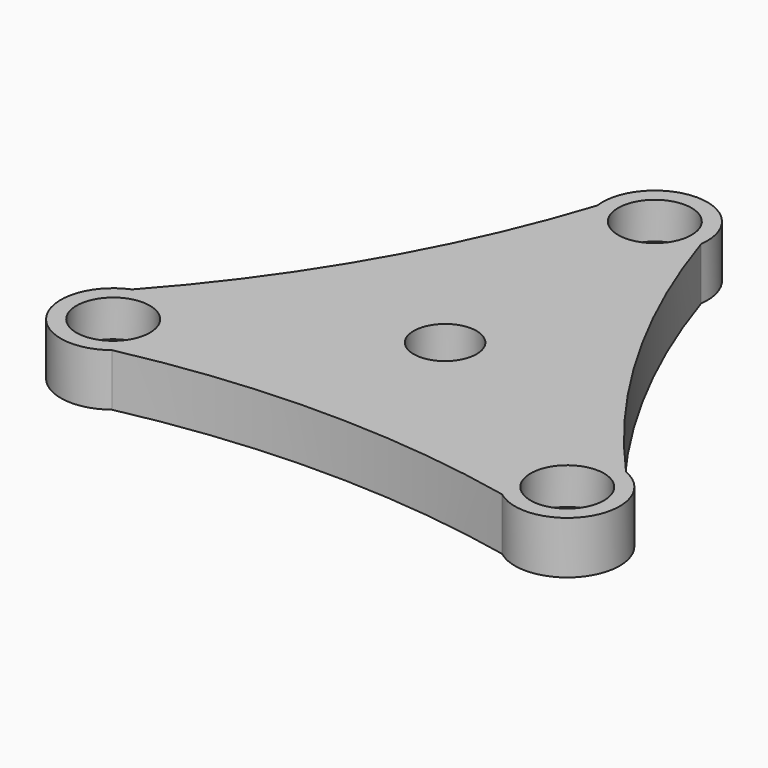
from build123d import *

# Parameters (mm, degrees)
F1_R     = 7
F1_R_2   = 6
F1_R_3   = 5
F2_DEPTH = 3
F3_DEPTH = 10


# Not quite as in the source:
# - a feature of the source that left no trace in its solid (it failed there, or was rolled back) is left out


with BuildPart() as f2:
    # F1 (on Top) → F2 (new body)
    with BuildSketch(Plane.XY):
        with BuildLine():
            ThreePointArc((9.9107145783, 48.6666821283), (0, 60), (-9.9107145783, 48.6666821283))
            ThreePointArc((-9.9107145783, 48.6666821283), (-25.1057988762, 14.4948397394), (-47.1019403302, -15.7504104697))
            ThreePointArc((-47.1019403302, -15.7504104697), (-51.9615242271, -30), (-37.1912257519, -32.9162716586))
            ThreePointArc((-37.1912257519, -32.9162716586), (0, -28.9896794788), (37.1912257519, -32.9162716586))
            ThreePointArc((37.1912257519, -32.9162716586), (51.9615242271, -30), (47.1019403302, -15.7504104697))
            ThreePointArc((47.1019403302, -15.7504104697), (25.1057988762, 14.4948397394), (9.9107145783, 48.6666821283))
        make_face()
        with Locations((-43.3012701892, -25)):
            Circle(F1_R, mode=Mode.SUBTRACT)
        with Locations((43.3012701892, -25)):
            Circle(F1_R, mode=Mode.SUBTRACT)
        Circle(F1_R_2, mode=Mode.SUBTRACT)
        with Locations((0, 50)):
            Circle(F1_R, mode=Mode.SUBTRACT)
        with Locations((-43.3012701892, -25)):
            Circle(F1_R)
        with Locations((-43.3012701892, -25)):
            Circle(F1_R_3, mode=Mode.SUBTRACT)
        with Locations((43.3012701892, -25)):
            Circle(F1_R)
        with Locations((43.3012701892, -25)):
            Circle(F1_R_3, mode=Mode.SUBTRACT)
        with Locations((0, 50)):
            Circle(F1_R)
        with Locations((0, 50)):
            Circle(F1_R_3, mode=Mode.SUBTRACT)
    extrude(amount=F2_DEPTH)

    # F1 (on Top) → F3 (join)
    with BuildSketch(Plane.XY):
        with BuildLine():
            ThreePointArc((9.9107145783, 48.6666821283), (0, 60), (-9.9107145783, 48.6666821283))
            ThreePointArc((-9.9107145783, 48.6666821283), (-25.1057988762, 14.4948397394), (-47.1019403302, -15.7504104697))
            ThreePointArc((-47.1019403302, -15.7504104697), (-51.9615242271, -30), (-37.1912257519, -32.9162716586))
            ThreePointArc((-37.1912257519, -32.9162716586), (0, -28.9896794788), (37.1912257519, -32.9162716586))
            ThreePointArc((37.1912257519, -32.9162716586), (51.9615242271, -30), (47.1019403302, -15.7504104697))
            ThreePointArc((47.1019403302, -15.7504104697), (25.1057988762, 14.4948397394), (9.9107145783, 48.6666821283))
        make_face()
        with Locations((-43.3012701892, -25)):
            Circle(F1_R, mode=Mode.SUBTRACT)
        with Locations((43.3012701892, -25)):
            Circle(F1_R, mode=Mode.SUBTRACT)
        Circle(F1_R_2, mode=Mode.SUBTRACT)
        with Locations((0, 50)):
            Circle(F1_R, mode=Mode.SUBTRACT)
    extrude(amount=F3_DEPTH)


solid = f2.part
